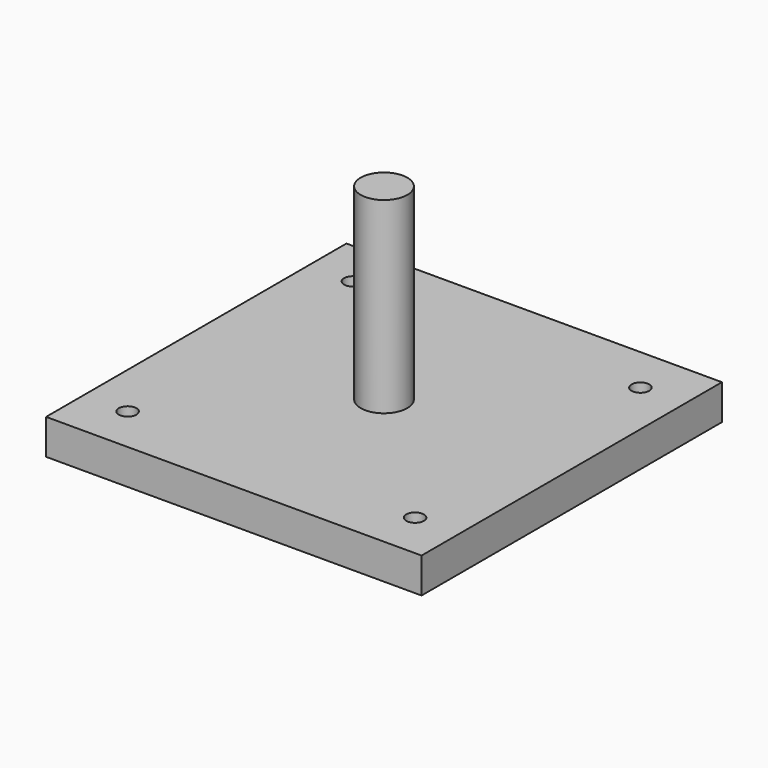
from build123d import *

# Parameters (mm, degrees)
F0_W     = 203.2
F0_H     = 203.2
F1_DEPTH = 19.05
F3_D     = 9.525
F4_R     = 12.6365
F5_DEPTH = 101.6


# Not quite as in the source:
# - a length typed as a fraction of an inch, garbled in the dataset ("3 / 203.2 mm" for 3/8 in), is restored


with BuildPart() as f1:
    # F0 (on Top) → F1 (new body)
    with BuildSketch(Plane.XY):
        Rectangle(F0_W, F0_H)
    extrude(amount=F1_DEPTH)

    # F3 (through all)
    with Locations(Plane.XY.offset(19.05)):
        with Locations((-77.7875, 76.2), (77.7875, 76.2), (-77.7875, -76.2), (77.7875, -76.2)):
            Hole(F3_D / 2)

    # F4 (on face) → F5 (join)
    with BuildSketch(Plane.XY.offset(19.05)):
        Circle(F4_R)
    extrude(amount=F5_DEPTH)


solid = f1.part
